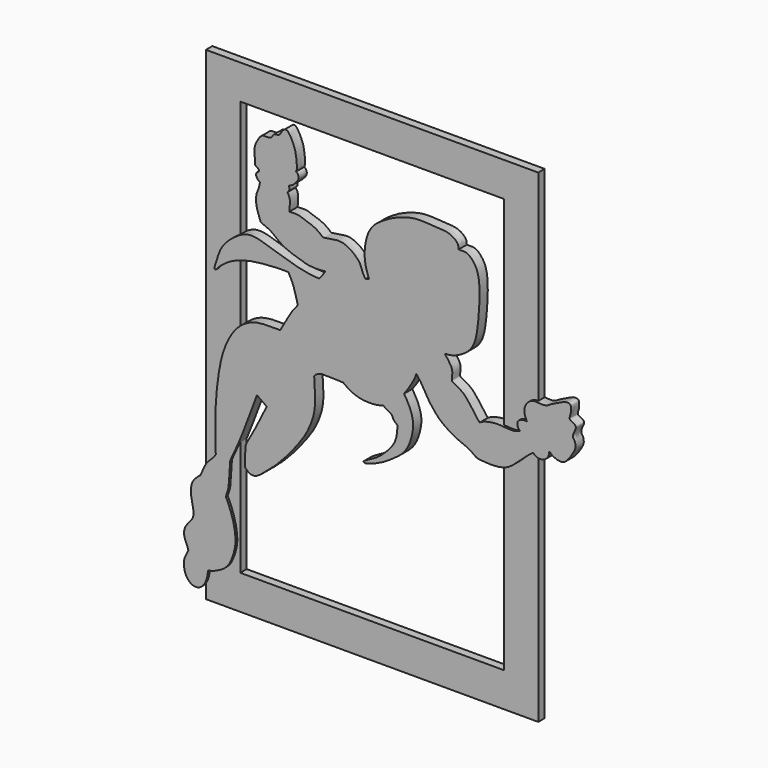
from build123d import *

# Parameters (mm, degrees)
F0_W     = 73.66
F0_H     = 107.188
F0_W_2   = 58.42
F0_H_2   = 91.948
F1_DEPTH = 1.778
F3_DEPTH = 2.286


# Not quite as in the source:
# - the program builds the solid bodies; features that only make, move or delete a surface that nothing else refers to are left out


with BuildPart() as f1:
    # F0 (on Front) → F1 (new body)
    with BuildSketch(Plane.XZ):
        Rectangle(F0_W, F0_H)
        Rectangle(F0_W_2, F0_H_2, mode=Mode.SUBTRACT)
    extrude(amount=F1_DEPTH)

    # F2 (on Front) → F3 (join)
    with BuildSketch(Plane.XZ):
        with BuildLine():
            add(Edge.make_bspline(
                [(-16.0454064608, 10.7553685084), (-16.5404903197, 10.1477843507), (-17.6103867163, 8.8347702237), (-19.0812257676, 6.0873701321), (-19.9224354692, 4.5540812934), (-20.1399513991, 4.5877092542), (-22.6988551585, 4.6587090133), (-25.4499731052, 4.423136561), (-27.4263655149, 3.579937367), (-29.695103518, 1.983974083), (-31.6924890789, -1.2233871876), (-33.2015282815, -5.2165342864), (-34.0304256877, -11.3971027055), (-34.4405058789, -16.1352578715), (-34.2596555248, -24.1201459803), (-34.2188760295, -24.3640903814), (-35.1217976189, -25.5447126262), (-36.6000700336, -26.6666106067), (-37.5915342494, -29.6505059275), (-38.0106073874, -29.641966975), (-39.031494438, -30.781801596), (-39.5690094309, -31.5164995115), (-39.9273296074, -33.7386112827), (-39.1576632172, -36.4188393786), (-39.1129730249, -38.3021200252), (-40.1045640427, -39.3253057857), (-41.1598790978, -40.7011690273), (-41.4311788322, -42.4185989883), (-40.5102389061, -44.2753905143), (-40.3570719235, -44.8111172404), (-40.2993187308, -45.0131185353)],
                knots=[0, 0, 0, 0, 0.0384369614, 0.08306384, 0.1130197561, 0.1223573728, 0.1600317707, 0.2023196761, 0.2374650076, 0.2774302962, 0.3242896965, 0.3752982991, 0.4347427393, 0.4934298642, 0.5594652492, 0.5712066747, 0.5984537303, 0.6344609503, 0.6755726218, 0.6900200078, 0.7189056168, 0.7430642882, 0.7785285288, 0.8201756613, 0.8524809122, 0.8807138533, 0.912497086, 0.9443709878, 0.9790245064, 1, 1, 1, 1], degree=3))
            add(Edge.make_bspline(
                [(-40.2993187308, -45.0131185353), (-40.4575826502, -45.3095447885), (-40.797498256, -45.946202277), (-41.4018194863, -47.2299823804), (-41.2624530421, -48.7390041685), (-40.9067798854, -50.2195722591), (-39.6012269612, -51.6259107722), (-38.0975019614, -51.6460596305), (-37.0788945174, -50.981398177), (-36.3040323557, -49.6518360353), (-36.0013232989, -48.2604090328), (-35.9936879743, -47.7379495281), (-35.9905250371, -47.521520406)],
                knots=[0, 0, 0, 0, 0.0891122151, 0.191393166, 0.2971142138, 0.4046702568, 0.5209819427, 0.6223870064, 0.7154638538, 0.823174928, 0.9267501217, 1, 1, 1, 1], degree=3))
            add(Edge.make_bspline(
                [(-35.9905250371, -47.521520406), (-35.5315747411, -47.4201638138), (-34.4467942768, -47.1805961478), (-31.7616817846, -45.7826177956), (-30.6479701622, -43.598557932), (-29.8154055634, -40.908693892), (-29.8577858095, -38.1896172201), (-30.62835519, -34.8590166694), (-31.7638111558, -32.2620632222), (-31.9688043547, -31.950575024), (-32.0256315172, -31.8642258644)],
                knots=[0, 0, 0, 0, 0.1040978049, 0.2460468294, 0.3762911289, 0.5142803063, 0.6511611107, 0.8098541763, 0.9472887507, 1, 1, 1, 1], degree=3))
            add(Edge.make_bspline(
                [(-32.0256315172, -31.8642258644), (-31.8273045831, -31.3302152369), (-31.4151967843, -30.2205830771), (-31.2813702608, -28.3946754603), (-31.1040045462, -25.1564102462), (-31.0332981699, -24.1603105789), (-29.5132077015, -21.2702354249), (-28.4330882301, -18.5871243956), (-27.1243560295, -15.2316155836), (-25.3043055787, -10.1670667104), (-25.1422079199, -9.8436739874), (-25.1093059778, -9.7780330107)],
                knots=[0, 0, 0, 0, 0.0938922139, 0.1951006491, 0.3229785167, 0.3977732902, 0.5243802869, 0.6486239992, 0.793557579, 0.9580971334, 1, 1, 1, 1], degree=3))
            add(Edge.make_bspline(
                [(-25.1093059778, -9.7780330107), (-24.7788596706, -9.9889989614), (-24.0861500535, -10.4312437067), (-23.339459115, -11.0075792811), (-22.9489654303, -11.3089829683)],
                knots=[0, 0, 0, 0, 0.4770343866, 1, 1, 1, 1], degree=3))
            add(Edge.make_bspline(
                [(-22.9489654303, -11.3089829683), (-23.1198105542, -11.6743517482), (-23.52288598, -12.536367433), (-24.6474990322, -14.6931083219), (-25.9798179455, -17.4276037697), (-27.4328021229, -19.7107703539), (-27.7331467169, -20.8539155603), (-27.7285282893, -22.4825767674), (-27.7263106396, -24.3857807641), (-27.8240491495, -24.6512172216), (-27.3015693096, -25.2132381081), (-26.5838623796, -25.7123844577), (-25.2958412846, -25.8624499033), (-22.7735775498, -23.7812764344), (-19.842316229, -21.1457800267), (-16.633111142, -17.3186236067), (-14.0803224302, -13.7811563774), (-12.3840606486, -9.7507865293), (-12.0871104252, -6.1359930054), (-12.4409500895, -2.0719937431), (-12.4109053586, -1.7655078109), (-11.2260773295, -0.9178082261), (-9.6478841459, -0.9905425844), (-6.6635253628, -1.0561354471), (-6.1632415533, -1.0915525136), (-6.0064583085, -1.1026518187)],
                knots=[0, 0, 0, 0, 0.0349013577, 0.0823428803, 0.1372340761, 0.1869059523, 0.2192090062, 0.259324265, 0.3008007961, 0.3157327968, 0.3408772497, 0.3696973561, 0.401873634, 0.4554616205, 0.5177213249, 0.5859390792, 0.6503434074, 0.7128481019, 0.7741709489, 0.8334071441, 0.8491309367, 0.8827625046, 0.9235361854, 0.9760371119, 1, 1, 1, 1], degree=3))
            add(Edge.make_bspline(
                [(-6.0064583085, -1.1026518187), (-5.5339666781, -1.46885947), (-4.4807531711, -2.2851593152), (-1.8086266643, -3.2239934332), (1.2296243122, -3.1739789109), (2.4156487886, -2.8552771169), (2.9240804724, -2.7186542284)],
                knots=[0, 0, 0, 0, 0.2244887724, 0.500399567, 0.7858284593, 1, 1, 1, 1], degree=3))
            add(Edge.make_bspline(
                [(2.9240804724, -2.7186542284), (3.2111325659, -2.947283306), (3.7748245651, -3.3962484409), (4.8393078404, -3.7381574764), (5.0902346283, -4.7993926529), (5.7323091452, -5.2858025497), (6.0710320249, -5.5424054153)],
                knots=[0, 0, 0, 0, 0.2527369206, 0.4963063614, 0.7342791915, 1, 1, 1, 1], degree=3))
            add(Edge.make_bspline(
                [(6.0710320249, -5.5424054153), (6.0306283379, -6.1210831311), (5.9491265139, -7.2883847533), (5.5193907242, -9.0710464081), (4.3206457983, -10.7219811454), (2.8929014673, -12.132944501), (1.317516412, -13.4997704416), (-1.3089683343, -14.7670753138), (-1.5420843505, -15.0830965461), (-1.0559303592, -15.3380646699), (-0.0895788516, -14.9982249736), (2.2622377999, -14.1849910009), (5.3743410584, -12.1703529045), (8.1349805449, -10.0278710006), (9.4002907244, -6.3387355004), (9.6651731303, -3.5067571994), (8.6088568035, -0.6289495359), (7.8347697045, 0.5656926598), (7.4829072692, 1.108719036)],
                knots=[0, 0, 0, 0, 0.0576772968, 0.1163459388, 0.178274009, 0.2392533467, 0.3055519251, 0.3788919864, 0.3994641024, 0.4264047845, 0.4691509039, 0.5378494533, 0.6226906318, 0.7041638292, 0.788463308, 0.8623735833, 0.9374417088, 1, 1, 1, 1], degree=3))
            add(Edge.make_bspline(
                [(7.4829072692, 1.108719036), (7.7756931484, 1.4840642756), (8.4475651108, 2.3453897719), (9.8016724211, 4.6410902952), (10.0875192842, 5.5141081447), (10.2045945823, 5.8716731146)],
                knots=[0, 0, 0, 0, 0.3131933958, 0.7187022203, 1, 1, 1, 1], degree=3))
            add(Edge.make_bspline(
                [(10.2045945823, 5.8716731146), (10.5404851135, 5.4736209651), (11.3085957244, 4.563359879), (12.7151027092, 1.9502449177), (13.0276867943, 1.4833057176), (13.1304105744, 1.3298565755)],
                knots=[0, 0, 0, 0, 0.342858621, 0.7840451586, 1, 1, 1, 1], degree=3))
            add(Edge.make_bspline(
                [(13.1304105744, 1.3298565755), (13.4078059917, 0.9601611226), (13.9679993074, 0.2135701243), (14.9052770231, -0.9309836426), (16.0615637925, -1.9742922899), (17.981951052, -3.2512442869), (20.0505149266, -4.2623271505), (21.7848884509, -4.8606340608), (22.9965898185, -5.7466028867), (23.4277121788, -6.0824649274), (24.0454740701, -6.3302752873), (26.8703679318, -6.531539714), (29.8165705466, -6.2635029936), (31.7908170608, -4.8986098042), (33.4753717252, -3.3284777451), (35.0719313595, -1.8235288978), (35.7657531427, -1.3174119486), (36.0601618886, -1.1026518187)],
                knots=[0, 0, 0, 0, 0.0598119331, 0.1207887479, 0.1838219719, 0.2607406957, 0.338092179, 0.4076120993, 0.468386722, 0.5042047224, 0.5429521244, 0.6272568673, 0.7157934736, 0.7925362031, 0.8701654267, 0.9449074174, 1, 1, 1, 1], degree=3))
            add(Edge.make_bspline(
                [(36.0601618886, -1.1026518187), (36.1948396624, -1.2035046167), (36.4811198989, -1.4178841842), (36.9931160515, -1.8804250606), (38.4052119434, -1.8466459248), (39.3930099631, -1.057989445), (39.5825580278, -0.3322022708), (39.6602825774, 0.0937902129), (39.6980009973, 0.3005172184)],
                knots=[0, 0, 0, 0, 0.1321665162, 0.2809421366, 0.4940502971, 0.6969769273, 0.8529479866, 1, 1, 1, 1], degree=3))
            add(Edge.make_bspline(
                [(39.6980009973, 0.3005172184), (39.9490870783, 0.0699781161), (40.3994931537, -0.3435701456), (40.994824069, -0.572978235), (41.5488733744, -0.8237370123), (42.8733718542, -0.9562915804), (44.0534908938, 0.2378771315), (45.392246071, 2.3559105046), (45.5589625791, 3.2075993793), (45.3425280765, 4.2559918865), (44.9434879431, 4.594269852), (44.9017806141, 5.3711155184), (45.4949364644, 6.4955253746), (45.6441557798, 7.0100049187), (45.3426507799, 7.4607608531), (44.541792687, 7.7843225082), (44.0227107329, 8.1809061161), (44.4761300068, 9.1335308625), (44.4994262726, 10.2918465196), (44.4498725464, 11.0611762355), (43.3919641645, 11.2846836596), (42.1072170284, 10.6222557891), (40.2951975259, 9.8518688445), (39.1347301197, 8.9723085546), (37.8497866685, 8.9647514691), (37.0603695191, 9.0011952005), (36.0003422191, 9.1445540009), (34.4774495564, 8.1630805924), (33.9940732213, 6.4141743617), (34.3959565593, 5.1814603983), (34.6340227643, 4.7474214402), (34.7350984812, 4.5631416142)],
                knots=[0, 0, 0, 0, 0.0334698849, 0.0600393278, 0.0865046637, 0.1234685925, 0.1675563901, 0.2212545022, 0.2534246553, 0.2871458323, 0.3108509592, 0.3395710839, 0.3783071216, 0.4023386942, 0.4256267546, 0.4576077543, 0.482438274, 0.5153919126, 0.5530528265, 0.5805156385, 0.6120460507, 0.6533586656, 0.7016131355, 0.7426796177, 0.7800567873, 0.8103874238, 0.8445379905, 0.8887766836, 0.9337931739, 0.9718905823, 1, 1, 1, 1], degree=3))
            add(Edge.make_bspline(
                [(34.7350984812, 4.5631416142), (34.4959195035, 4.5798657001), (33.9895509193, 4.6152724561), (33.0620246633, 4.3428193681), (32.587569887, 3.8333069091), (32.5524158313, 2.9702977076), (33.0333044863, 2.302786349), (33.1440300049, 2.2250508053), (33.178281039, 2.2010046523)],
                knots=[0, 0, 0, 0, 0.179404261, 0.3798188392, 0.546160113, 0.7345189176, 0.9178779948, 1, 1, 1, 1], degree=3))
            add(Edge.make_bspline(
                [(33.178281039, 2.2010046523), (32.9229067055, 2.1097298036), (32.4147804236, 1.9281173882), (31.6723042532, 1.668623734), (29.4046610911, 1.8563122867), (27.4526745787, 2.0272594146), (24.9880713658, 1.4260768914), (24.4308962359, 1.0418370492), (24.2214705795, 0.897412654)],
                knots=[0, 0, 0, 0, 0.1229844007, 0.2447059005, 0.4491245379, 0.6532919475, 0.8696826948, 1, 1, 1, 1], degree=3))
            add(Edge.make_bspline(
                [(24.2214705795, 0.897412654), (23.9328966895, 1.3069835936), (23.2895800921, 2.2200384207), (21.826169429, 4.1681378356), (20.5529582269, 5.7367025709), (18.7501494084, 6.5963916996), (18.2079605879, 6.9185969861), (18.0301809963, 7.1767166592), (18.176740709, 8.2553000048), (18.2486045821, 9.5311216499), (17.1828466055, 10.9956726807), (16.732879511, 11.5965531778), (16.5344253182, 11.8615664542)],
                knots=[0, 0, 0, 0, 0.110580147, 0.2465158713, 0.3736714173, 0.4953592011, 0.5614728408, 0.6054631581, 0.6934175962, 0.7937057773, 0.9090156726, 1, 1, 1, 1], degree=3))
            add(Edge.make_bspline(
                [(16.5344253182, 11.8615664542), (16.9925247323, 11.8799077452), (18.0482892215, 11.9221782286), (20.3932770765, 12.8800394856), (22.4086120743, 14.5131359608), (23.5111634956, 16.9604279561), (24.0113372421, 21.0549726349), (24.3205430159, 25.9261929402), (24.0653428751, 29.7216665977), (23.1122135991, 31.7024714241), (21.6036156084, 33.2492327676), (20.2590219227, 33.1726893247), (19.7739664216, 33.1799383435), (19.568786025, 33.1830047071)],
                knots=[0, 0, 0, 0, 0.0711810464, 0.1640482803, 0.2577768372, 0.3517052381, 0.4709711402, 0.6032922008, 0.7166690349, 0.8031489539, 0.8864261676, 0.9519578194, 1, 1, 1, 1], degree=3))
            add(Edge.make_bspline(
                [(19.568786025, 33.1830047071), (19.55112943, 33.5228300402), (19.5138465504, 34.2403900741), (18.5254874254, 35.194429538), (16.9403800659, 35.9027433847), (13.4011641361, 36.0215745539), (9.9459535721, 36.2279334707), (7.2515934538, 35.4843459334), (4.6396849682, 34.5116878101), (2.077612021, 32.9045721918), (0.7212975208, 31.8071579198), (-0.6009721043, 29.9683694193), (-1.2598102868, 26.9550553415), (-1.2859695296, 24.6518939936), (-0.877128136, 22.5611294315), (-0.4688778983, 21.4907618269), (-0.2759284107, 20.9848787636)],
                knots=[0, 0, 0, 0, 0.0477096292, 0.1007415276, 0.1624648404, 0.2517922316, 0.3412110177, 0.4195704992, 0.4995525062, 0.5815462363, 0.6439183755, 0.7140385027, 0.7972597364, 0.870065774, 0.9385897667, 1, 1, 1, 1], degree=3))
            add(Edge.make_bspline(
                [(-0.2759284107, 20.9848787636), (-0.4028283486, 20.9291007284), (-0.6583830685, 20.8167733277), (-0.9287501756, 20.7267589415), (-1.0648620082, 20.6814426929)],
                knots=[0, 0, 0, 0, 0.496566598, 1, 1, 1, 1], degree=3))
            add(Edge.make_bspline(
                [(-1.0648620082, 20.6814426929), (-1.2943340245, 21.0505263548), (-1.7762881948, 21.8257032713), (-2.1220082007, 23.423211573), (-3.8111056493, 25.0953314961), (-5.5395227452, 26.0325279574), (-6.9845330355, 26.3270562455), (-8.9471765246, 26.0141591899), (-10.1994028367, 25.8202256562), (-10.4528261718, 25.6717462718), (-10.9441268561, 26.2322345154), (-12.5150822577, 27.3095694628), (-14.5831716706, 27.8416933015), (-15.8466566587, 28.4643984527), (-17.3089535559, 28.354115717), (-17.744408747, 28.3644296249), (-17.9156735539, 28.3684860915)],
                knots=[0, 0, 0, 0, 0.0702625578, 0.1475706419, 0.2412388314, 0.3268173731, 0.4004184695, 0.4883398642, 0.5559154066, 0.5837709786, 0.6314141664, 0.7169927272, 0.8073160271, 0.8805661044, 0.953026572, 1, 1, 1, 1], degree=3))
            add(Edge.make_bspline(
                [(-17.9156735539, 28.3684860915), (-17.8819443804, 28.7593040547), (-17.8105643598, 29.5863801822), (-17.7831381583, 31.1865889628), (-18.1926345445, 31.7423750263), (-18.3722730726, 31.9861881435)],
                knots=[0, 0, 0, 0, 0.3345985089, 0.7081006122, 1, 1, 1, 1], degree=3))
            add(Edge.make_bspline(
                [(-18.3722730726, 31.9861881435), (-18.2580881173, 32.0963729651), (-18.0222912662, 32.3239093678), (-17.8523736184, 32.8857878705), (-17.9899410071, 33.2300780502), (-18.0587247014, 33.40222314)],
                knots=[0, 0, 0, 0, 0.3194800248, 0.6597400124, 1, 1, 1, 1], degree=3))
            add(Edge.make_bspline(
                [(-18.0587247014, 33.40222314), (-17.7529881008, 33.5249878201), (-17.129627687, 33.7752903406), (-16.4011139904, 34.5956125492), (-15.8662955084, 35.198591739), (-15.8646904898, 36.2155005981), (-16.2577486466, 36.517763961), (-16.4415724576, 36.6591252387)],
                knots=[0, 0, 0, 0, 0.2120872872, 0.4324206484, 0.6229538492, 0.8236646177, 1, 1, 1, 1], degree=3))
            add(Edge.make_bspline(
                [(-16.4415724576, 36.6591252387), (-16.3624087711, 36.8593732794), (-16.1455273637, 37.4079843769), (-16.4386634164, 39.781707377), (-16.7432281764, 41.3881972819), (-17.9407651736, 43.7172931234), (-18.5482793152, 44.1673783259), (-19.1096670877, 44.0666513472), (-19.7295017201, 43.3043907996), (-20.0132725883, 42.7292970829), (-20.4895622217, 42.4098205186), (-21.1877762539, 42.5226692956), (-21.5790227609, 42.096569155), (-21.7987951133, 41.6523141439), (-22.1441317832, 41.3988121087), (-23.053784522, 41.3052885072), (-24.0613062953, 41.3591055861), (-24.7242617353, 40.4615501019), (-25.3337644415, 39.3854900285), (-25.6955516979, 38.4374735373), (-25.6375321104, 36.5940566694), (-25.5531371456, 35.1489086659), (-25.5130946606, 34.9051903051), (-24.6291817299, 34.4018988645), (-24.6072091545, 34.2416931326), (-24.6409276615, 33.9151710397), (-25.2578473571, 33.7944149548), (-25.3222432983, 33.0495554946), (-25.1511312558, 32.5667664052), (-24.6684765506, 32.0916843693), (-24.5122070075, 31.9861993443), (-24.4522839785, 31.9457501173)],
                knots=[0, 0, 0, 0, 0.0336627335, 0.0922243689, 0.1454002114, 0.2069994234, 0.2386622431, 0.2654643675, 0.303508622, 0.3349788525, 0.3629055269, 0.394225198, 0.4225291027, 0.4495108405, 0.4738539867, 0.51066849, 0.5486958426, 0.5881219533, 0.6312347682, 0.6700383466, 0.7238824507, 0.7694818945, 0.7886853576, 0.8264040911, 0.8416497712, 0.8612980014, 0.8895090119, 0.9206529333, 0.9491297572, 0.9804933259, 1, 1, 1, 1], degree=3))
            add(Edge.make_bspline(
                [(-24.4522839785, 31.9457501173), (-24.5164450353, 31.5525527016), (-24.6523555708, 30.7196538372), (-25.3910158619, 29.4054226164), (-25.2959936943, 27.1543789371), (-24.9013004409, 26.0040567779), (-24.4618866755, 24.7454793274), (-24.2622883464, 24.1972694025), (-23.5093109, 23.923039196), (-21.8728998948, 23.2509344187), (-20.6241862255, 22.0428104327), (-18.6519583294, 20.7879662199), (-15.6570711056, 19.8261298198), (-13.7947092401, 19.2152282651), (-11.4502088542, 19.1356499769), (-10.4132366263, 19.2508889344), (-9.9480422214, 19.3025860935)],
                knots=[0, 0, 0, 0, 0.0618107658, 0.1309319812, 0.2138635794, 0.2781463703, 0.3420683867, 0.3829033337, 0.4308579906, 0.505350234, 0.579792445, 0.6660530518, 0.7656686795, 0.846011522, 0.9309194822, 1, 1, 1, 1], degree=3))
            add(Edge.make_bspline(
                [(-9.9480422214, 19.3025860935), (-10.2235428589, 18.8727050348), (-10.7153275226, 18.1053423391), (-11.1518624471, 17.6442825568), (-11.3438479602, 17.4415111542)],
                knots=[0, 0, 0, 0, 0.5602058337, 1, 1, 1, 1], degree=3))
            add(Edge.make_bspline(
                [(-11.3438479602, 17.4415111542), (-12.1470630771, 17.4962641857), (-13.9804978695, 17.621244544), (-18.0520002067, 18.6385432086), (-22.3142523594, 20.1376608794), (-25.3486471511, 20.9990073729), (-27.3671336731, 20.998884694), (-29.1684281154, 20.1299830267), (-31.0645148085, 18.7424199626), (-32.7670045286, 16.9450761471), (-33.5636553174, 15.2499293941), (-34.2311260932, 13.038379555), (-34.5468504339, 12.1198665335), (-34.5412726017, 11.7613937855), (-34.1329107352, 11.6892927355), (-33.7558771122, 12.4290628782), (-31.5352821002, 14.1981079845), (-29.4424337179, 15.1426126294), (-26.2692797992, 16.1777328874), (-20.1518217866, 16.5978480858), (-18.6799736692, 16.5249165582), (-18.1508492678, 16.4986979216)],
                knots=[0, 0, 0, 0, 0.0569308554, 0.1299515023, 0.2067754451, 0.2695014449, 0.3185499751, 0.3678367064, 0.4227859408, 0.4781062838, 0.5274762149, 0.5816721683, 0.6162917723, 0.6346370524, 0.6529822593, 0.6830717005, 0.7424740932, 0.7967039732, 0.862482105, 0.9505627836, 1, 1, 1, 1], degree=3))
            add(Edge.make_bspline(
                [(-18.1508492678, 16.4986979216), (-17.8589926414, 15.982371139), (-17.2747187314, 14.9487257086), (-16.7221589666, 13.263437273), (-16.2855320327, 11.6452823858), (-16.0454064608, 10.7553685084)],
                knots=[0, 0, 0, 0, 0.3099551621, 0.6205057487, 1, 1, 1, 1], degree=3))
        make_face()
    extrude(amount=F3_DEPTH)


solid = f1.part
